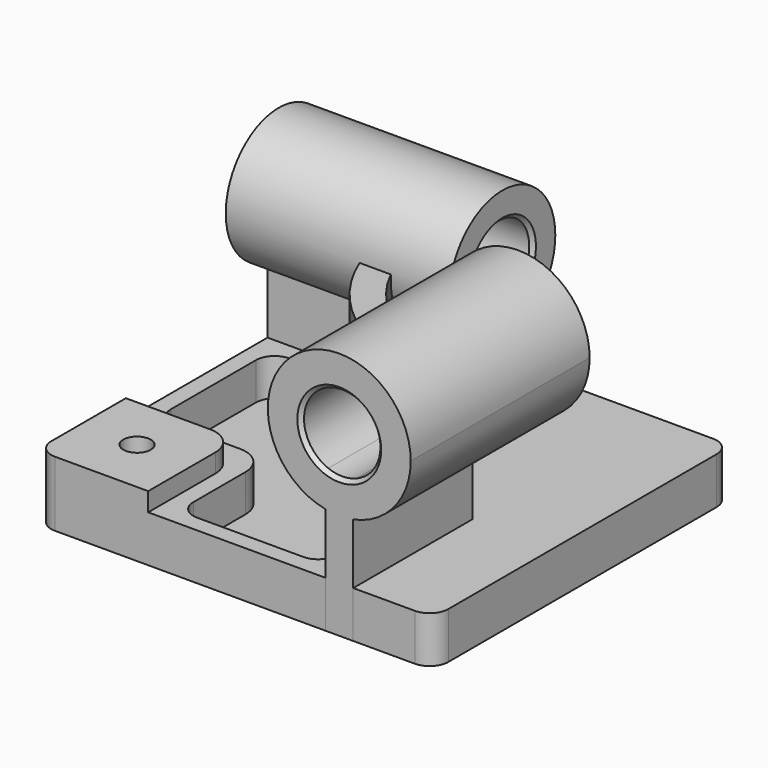
from build123d import *
from build123d import SkipClean  # not in build123d's __all__

# Parameters (mm, degrees)
F1_DEPTH       = 35
F2_DEPTH       = 25
F3_DEPTH       = 95
F4_DEPTH       = 5
F5_D           = 14.75
F5_CBORE_D     = 22.25
F5_CBORE_DEPTH = 14
F7_DEPTH       = 120
F8_DEPTH       = 120
F10_DEPTH      = 120
F11_DEPTH      = 120
F12_T2_ANGLE   = 42.9202554989
F12_T4_ANGLE   = 248.5398722506
F12_T6_ANGLE   = 68.5398722506


# Not quite as in the source:
# - a fillet or chamfer that OpenCascade refuses, or shapes differently, is made with other operations: its cross-section is extruded or revolved along the edge and cut away or added


with BuildPart() as f1:
    # F0 (on Top) → F1 (new body)
    with BuildSketch(Plane.XY):
        with BuildLine():
            Line((-96.5, -100), (-46.5, -100))
            Line((-46.5, -100), (-46.5, -55))
            ThreePointArc((-46.5, -55), (-50.8933982822, -44.3933982822), (-61.5, -40))
            Line((-61.5, -40), (-106.5, -40))
            Line((-106.5, -40), (-106.5, -90))
            ThreePointArc((-106.5, -90), (-103.5710678119, -97.0710678119), (-96.5, -100))
        make_face()
    extrude(amount=F1_DEPTH)

    # F0 (on Top) → F2 (join)
    with BuildSketch(Plane.XY):
        with BuildLine():
            Line((-46.5, -100), (48.5, -100))
            Line((48.5, -100), (48.5, -35))
            ThreePointArc((48.5, -35), (-12.7295911164, -6.2295911164), (-41.5, 55))
            Line((-41.5, 55), (-106.5, 55))
            Line((-106.5, 55), (-106.5, -40))
            Line((-106.5, -40), (-61.5, -40))
            ThreePointArc((-61.5, -40), (-50.8933982822, -44.3933982822), (-46.5, -55))
            Line((-46.5, -55), (-46.5, -100))
        make_face()
        with BuildLine():
            Line((-97.5, -21), (-97.5, 36))
            ThreePointArc((-97.5, 36), (-94.5710678119, 43.0710678119), (-87.5, 46))
            Line((-87.5, 46), (-60.5, 46))
            ThreePointArc((-60.5, 46), (-53.4289321881, 43.0710678119), (-50.5, 36))
            Line((-50.5, 36), (-50.5, 35.8177255686))
            ThreePointArc((-50.5, 35.8177255686), (-19.0382464985, -12.6488819399), (29.5, -44))
            ThreePointArc((29.5, -44), (36.5710678119, -46.9289321881), (39.5, -54))
            Line((39.5, -54), (39.5, -81))
            ThreePointArc((39.5, -81), (36.5710678119, -88.0710678119), (29.5, -91))
            Line((29.5, -91), (-27.5, -91))
            ThreePointArc((-27.5, -91), (-34.5710678119, -88.0710678119), (-37.5, -81))
            Line((-37.5, -81), (-37.5, -46))
            ThreePointArc((-37.5, -46), (-41.8933982822, -35.3933982822), (-52.5, -31))
            Line((-52.5, -31), (-87.5, -31))
            ThreePointArc((-87.5, -31), (-94.5710678119, -28.0710678119), (-97.5, -21))
        make_face(mode=Mode.SUBTRACT)
    extrude(amount=F2_DEPTH)

    # F0 (on Top) → F4 (join)
    with BuildSketch(Plane.XY):
        with BuildLine():
            ThreePointArc((-87.5, 46), (-94.5710678119, 43.0710678119), (-97.5, 36))
            Line((-97.5, 36), (-97.5, -21))
            ThreePointArc((-97.5, -21), (-94.5710678119, -28.0710678119), (-87.5, -31))
            Line((-87.5, -31), (-52.5, -31))
            ThreePointArc((-52.5, -31), (-41.8933982822, -35.3933982822), (-37.5, -46))
            Line((-37.5, -46), (-37.5, -81))
            ThreePointArc((-37.5, -81), (-34.5710678119, -88.0710678119), (-27.5, -91))
            Line((-27.5, -91), (29.5, -91))
            ThreePointArc((29.5, -91), (36.5710678119, -88.0710678119), (39.5, -81))
            Line((39.5, -81), (39.5, -54))
            ThreePointArc((39.5, -54), (36.5710678119, -46.9289321881), (29.5, -44))
            ThreePointArc((29.5, -44), (-19.0382464985, -12.6488819399), (-50.5, 35.8177255686))
            Line((-50.5, 35.8177255686), (-50.5, 36))
            ThreePointArc((-50.5, 36), (-53.4289321881, 43.0710678119), (-60.5, 46))
            Line((-60.5, 46), (-87.5, 46))
        make_face()
    extrude(amount=F4_DEPTH)

    # F5 (through all)
    with Locations(Plane(origin=(0, 0, 0), x_dir=(1, 0, 0), z_dir=(0, 0, -1))):
        with Locations((-76.5, 70)):
            CounterBoreHole(F5_D / 2, F5_CBORE_D / 2, F5_CBORE_DEPTH)


with BuildPart() as f2:
    # F0 (on Top) → F2, piece 2 (new body)
    with BuildSketch(Plane.XY):
        with BuildLine():
            Line((63.5, -100), (96.5, -100))
            ThreePointArc((96.5, -100), (103.5710678119, -97.0710678119), (106.5, -90))
            Line((106.5, -90), (106.5, 90))
            ThreePointArc((106.5, 90), (103.5710678119, 97.0710678119), (96.5, 100))
            Line((96.5, 100), (-96.5, 100))
            ThreePointArc((-96.5, 100), (-103.5710678119, 97.0710678119), (-106.5, 90))
            Line((-106.5, 90), (-106.5, 70))
            Line((-106.5, 70), (-26.5, 70))
            ThreePointArc((-26.5, 70), (-1.9204107639, 4.5795892361), (63.5, -20))
            Line((63.5, -20), (63.5, -100))
        make_face()
    extrude(amount=F2_DEPTH)


with BuildPart() as f3:
    # F0 (on Top) → F3 (new body)
    with BuildSketch(Plane.XY):
        with BuildLine():
            Line((48.5, -100), (63.5, -100))
            Line((63.5, -100), (63.5, -20))
            ThreePointArc((63.5, -20), (-1.9204107639, 4.5795892361), (-26.5, 70))
            Line((-26.5, 70), (-106.5, 70))
            Line((-106.5, 70), (-106.5, 55))
            Line((-106.5, 55), (-41.5, 55))
            ThreePointArc((-41.5, 55), (-12.7295911164, -6.2295911164), (48.5, -35))
            Line((48.5, -35), (48.5, -100))
        make_face()
    extrude(amount=F3_DEPTH)

    # F6 (on face) → F7 (cut)
    with BuildSketch(Plane.XZ.offset(100)):
        with BuildLine():
            Line((63.5, 75.9212159717), (63.5, 95))
            Line((63.5, 95), (48.5, 95))
            Line((48.5, 95), (48.5, 75.9212159717))
            ThreePointArc((48.5, 75.9212159717), (56, 74.5), (63.5, 75.9212159717))
        make_face()
        with BuildLine():
            Line((48.5, 95), (63.5, 95))
            Line((63.5, 95), (63.5, 75.9212159717))
            ThreePointArc((63.5, 75.9212159717), (72.9410743461, 83.4566036194), (76.5, 95))
            ThreePointArc((76.5, 95), (44.4566036194, 111.9410743461), (48.5, 75.9212159717))
            Line((48.5, 75.9212159717), (48.5, 95))
        make_face()
    extrude(amount=-F7_DEPTH, mode=Mode.SUBTRACT)

    # F6 (on face) → F8 (join)
    with BuildSketch(Plane.XZ.offset(100)):
        with BuildLine():
            ThreePointArc((76.5, 95), (72.9410743461, 83.4566036194), (63.5, 75.9212159717))
            Line((63.5, 75.9212159717), (63.5, 57.4075214209))
            ThreePointArc((63.5, 57.4075214209), (85.6390320848, 70.6900797451), (94.33333335, 95))
            ThreePointArc((94.33333335, 95), (31.6900797451, 124.6390320848), (48.5, 57.4075214209))
            Line((48.5, 57.4075214209), (48.5, 75.9212159717))
            ThreePointArc((48.5, 75.9212159717), (44.4566036194, 111.9410743461), (76.5, 95))
        make_face()
        with BuildLine():
            Line((63.5, 57.4075214209), (63.5, 75.9212159717))
            ThreePointArc((63.5, 75.9212159717), (56, 74.5), (48.5, 75.9212159717))
            Line((48.5, 75.9212159717), (48.5, 57.4075214209))
            ThreePointArc((48.5, 57.4075214209), (56, 56.66666665), (63.5, 57.4075214209))
        make_face()
    extrude(amount=-F8_DEPTH)

    # F9 (on face) → F10 (cut)
    with BuildSketch(Plane(origin=(-106.5, 0, 0), x_dir=(0, -1, 0), z_dir=(-1, 0, 0))):
        with BuildLine():
            Line((-55, 75.9212159717), (-55, 95))
            Line((-55, 95), (-70, 95))
            Line((-70, 95), (-70, 75.9212159717))
            ThreePointArc((-70, 75.9212159717), (-62.5, 74.5), (-55, 75.9212159717))
        make_face()
        with BuildLine():
            Line((-70, 95), (-55, 95))
            Line((-55, 95), (-55, 75.9212159717))
            ThreePointArc((-55, 75.9212159717), (-45.5589256539, 83.4566036194), (-42, 95))
            ThreePointArc((-42, 95), (-74.0433963806, 111.9410743461), (-70, 75.9212159717))
            Line((-70, 75.9212159717), (-70, 95))
        make_face()
    extrude(amount=-F10_DEPTH, mode=Mode.SUBTRACT)

    # F9 (on face) → F11 (join)
    with BuildSketch(Plane(origin=(-106.5, 0, 0), x_dir=(0, -1, 0), z_dir=(-1, 0, 0))):
        with BuildLine():
            ThreePointArc((-42, 95), (-45.5589256539, 83.4566036194), (-55, 75.9212159717))
            Line((-55, 75.9212159717), (-55, 60.3012968542))
            ThreePointArc((-55, 60.3012968542), (-34.8730204329, 72.7065031904), (-27, 95))
            ThreePointArc((-27, 95), (-84.7934968096, 122.6269795671), (-70, 60.3012968542))
            Line((-70, 60.3012968542), (-70, 75.9212159717))
            ThreePointArc((-70, 75.9212159717), (-74.0433963806, 111.9410743461), (-42, 95))
        make_face()
        with BuildLine():
            Line((-55, 60.3012968542), (-55, 75.9212159717))
            ThreePointArc((-55, 75.9212159717), (-62.5, 74.5), (-70, 75.9212159717))
            Line((-70, 75.9212159717), (-70, 60.3012968542))
            ThreePointArc((-70, 60.3012968542), (-62.5, 59.5), (-55, 60.3012968542))
        make_face()
    with SkipClean():  # cleaning this boolean's faces spoils the solid; the shape is the same uncleaned
        extrude(amount=-F11_DEPTH)

    # F12: chamfer of 2 on 6 edges, made by hand

    # F12_s1 → F12_t2 (revolve, cut)
    with BuildSketch(Plane(origin=(0, 86.4809842241, 33.9962641601), x_dir=(1, 0, 0), z_dir=(0, 0.9306723916, 0.3658536585))):
        Polygon((-106.5, -43.048023546), (-104.5, -45.048023546), (-106.5, -45.048023546), align=None)
    revolve(axis=Axis((-106.5, 62.5, 95), (-1, 0, 0)), revolution_arc=F12_T2_ANGLE, mode=Mode.SUBTRACT)

    # F12_s3 → F12_t4 (revolve, cut)
    with BuildSketch(Plane(origin=(0, 86.4809842241, 33.9962641601), x_dir=(1, 0, 0), z_dir=(0, -0.9306723916, -0.3658536585))):
        Polygon((-106.5, 43.048023546), (-104.5, 45.048023546), (-106.5, 45.048023546), align=None)
    revolve(axis=Axis((-106.5, 62.5, 95), (1, 0, 0)), revolution_arc=F12_T4_ANGLE, mode=Mode.SUBTRACT)

    # F12_s5 → F12_t6 (revolve, cut)
    with BuildSketch(Plane.XY.offset(95)):
        Polygon((-106.5, 40), (-104.5, 42), (-106.5, 42), align=None)
    revolve(axis=Axis((-106.5, 62.5, 95), (1, 0, 0)), revolution_arc=F12_T6_ANGLE, mode=Mode.SUBTRACT)

    # F12_s7 → F12_t8 (revolve, cut)
    with BuildSketch(Plane.XY.offset(95)):
        Polygon((13.5, 40), (11.5, 42), (13.5, 42), align=None)
    revolve(axis=Axis((13.5, 62.5, 95), (1, 0, 0)), mode=Mode.SUBTRACT)

    # F12_s9 → F12_t10 (revolve, cut)
    with BuildSketch(Plane.XY.offset(95)):
        Polygon((76.5, 18), (78.5, 20), (76.5, 20), align=None)
    revolve(axis=Axis((56, 20, 95), (0, 1, 0)), mode=Mode.SUBTRACT)

    # F12_s11 → F12_t12 (revolve, cut)
    with BuildSketch(Plane.XY.offset(95)):
        Polygon((78.5, -100), (76.5, -98), (76.5, -100), align=None)
    revolve(axis=Axis((56, -100, 95), (0, 1, 0)), mode=Mode.SUBTRACT)


solid = Compound([f1.part, f2.part, f3.part])
